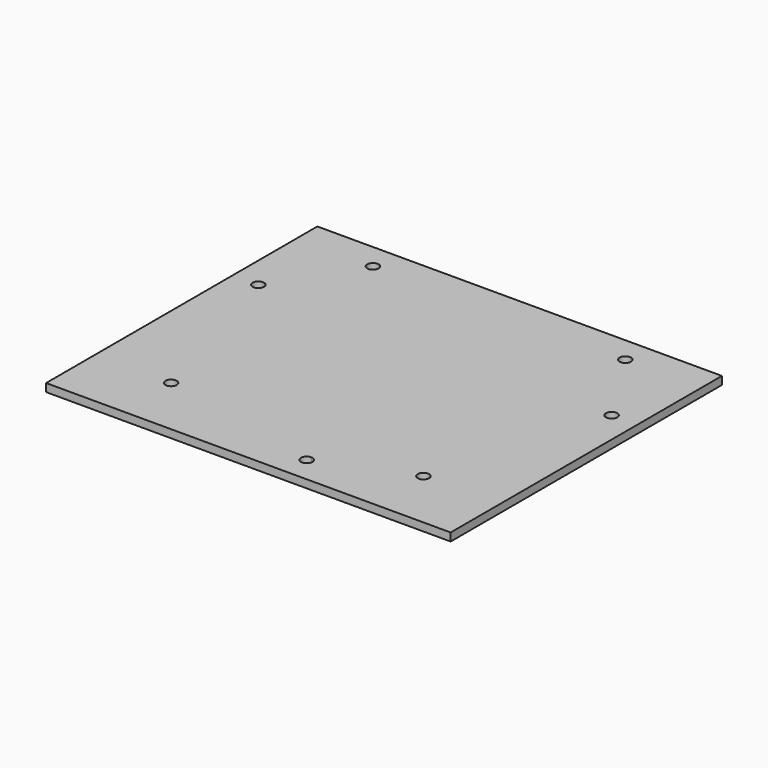
from build123d import *

# Parameters (mm, degrees)
F0_W     = 160.32
F0_H     = 134.37
F0_R     = 2.25
F1_DEPTH = 3.175


# Not quite as in the source:
# - a length typed as a fraction of an inch, garbled in the dataset ("3 / 203.2 mm" for 3/8 in), is restored


with BuildPart() as f1:
    # F0 (on Top) → F1 (new body)
    with BuildSketch(Plane.XY):
        with Locations((-15, 57.025)):
            Rectangle(F0_W, F0_H)
        with Locations((-65, 14.05)):
            Circle(F0_R, mode=Mode.SUBTRACT)
        with BuildLine():
            ThreePointArc((0, 2.25), (1.5909902577, 1.5909902577), (2.25, 0))
            ThreePointArc((2.25, 0), (-1.5909902577, -1.5909902577), (0, 2.25))
        make_face(mode=Mode.SUBTRACT)
        with Locations((35, 14.05)):
            Circle(F0_R, mode=Mode.SUBTRACT)
        with Locations((-85, 82.3)):
            Circle(F0_R, mode=Mode.SUBTRACT)
        with Locations((-65, 114.05)):
            Circle(F0_R, mode=Mode.SUBTRACT)
        with Locations((55, 82.3)):
            Circle(F0_R, mode=Mode.SUBTRACT)
        with Locations((35, 114.05)):
            Circle(F0_R, mode=Mode.SUBTRACT)
    extrude(amount=F1_DEPTH)


solid = f1.part
